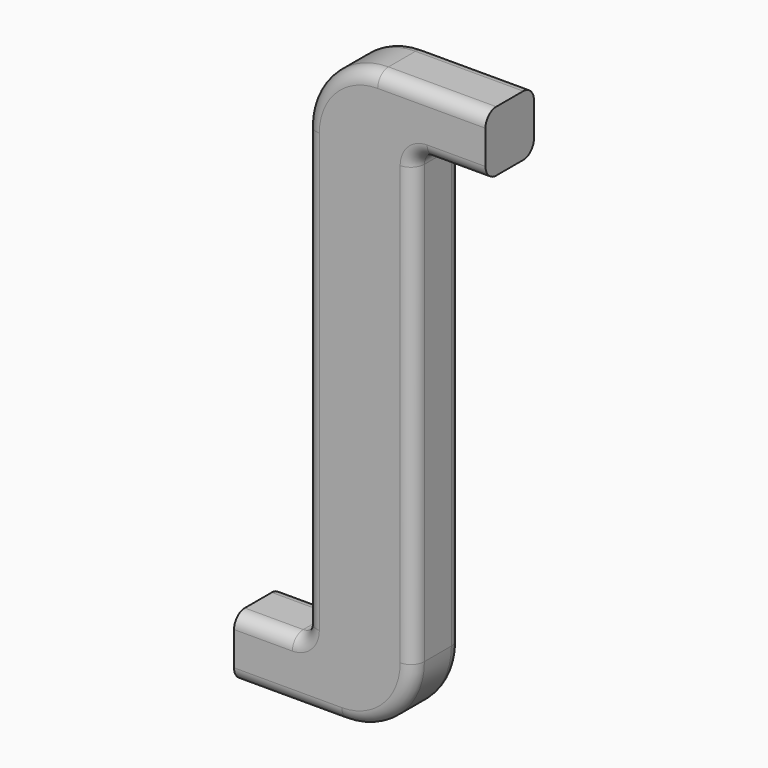
from build123d import *

# Parameters (mm, degrees)
F1_DEPTH = 6.75
F2_R     = 8
F3_R     = 1.5


with BuildPart() as f1:
    # F0 (on Front) → F1 (new body)
    with BuildSketch(Plane.XZ):
        Polygon((-90.6164456464, 33.1331632659), (-102.6164456464, 33.1331632659), (-102.6164456464, 26.3831632659), (-102.6164456464, -25.1168367341), (-110.6164456464, -25.1168367341), (-110.6164456464, -31.8668367341), (-102.6164456464, -31.8668367341), (-90.6164456464, -31.8668367341), (-90.6164456464, -25.1168367341), (-90.6164456464, 26.3831632659), (-82.6164456464, 26.3831632659), (-82.6164456464, 33.1331632659), align=None)
    extrude(amount=F1_DEPTH)

    # F2
    f2_edges = [f1.edges().sort_by_distance(p)[0] for p in [
        (-102.616446, -3.375, 33.133163),
        (-90.616446, -3.375, -31.866837),
    ]]
    fillet(f2_edges, radius=F2_R)

    # F3
    f3_edges = [f1.edges().sort_by_distance(p)[0] for p in [
        (-102.616446, 0, 0.008163),
        (-106.616446, 0, -25.116837),
        (-102.616446, -6.75, 0.008163),
        (-106.616446, -6.75, -25.116837),
        (-102.616446, -3.375, -25.116837),
        (-104.616446, -6.75, -31.866837),
        (-104.616446, 0, -31.866837),
        (-90.616446, -3.375, 26.383163),
        (-100.2733, 0, 30.790018),
        (-88.616446, 0, 33.133163),
        (-86.616446, 0, 26.383163),
        (-92.959591, 0, -29.523691),
        (-90.616446, 0, 1.258163),
        (-100.2733, -6.75, 30.790018),
        (-88.616446, -6.75, 33.133163),
        (-86.616446, -6.75, 26.383163),
        (-92.959591, -6.75, -29.523691),
        (-90.616446, -6.75, 1.258163),
    ]]
    fillet(f3_edges, radius=F3_R)


solid = f1.part
